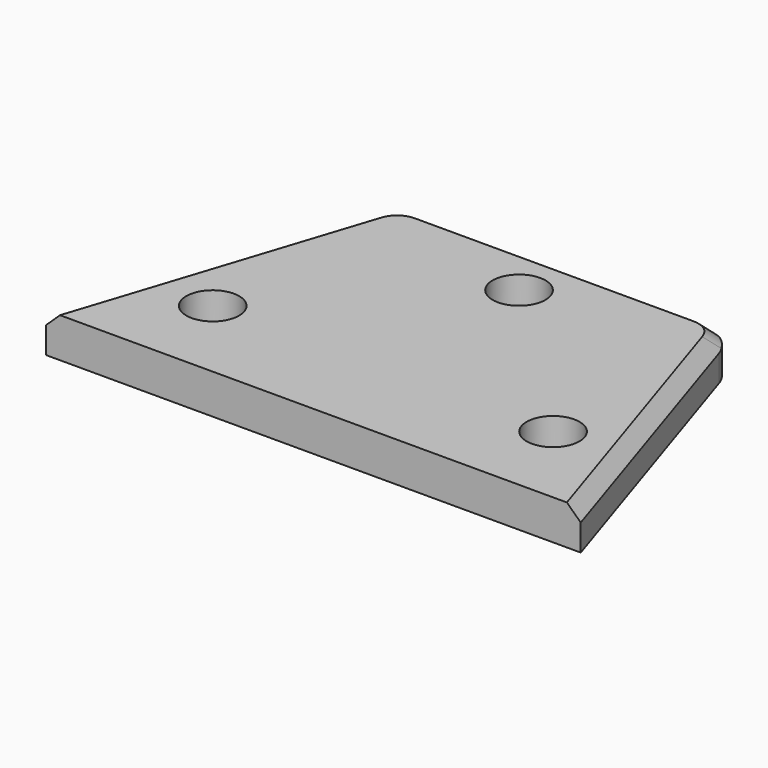
from build123d import *

# Parameters (mm, degrees)
F0_R     = 4
F1_DEPTH = 6
F2_SIZE  = 2
F3_F1_R  = 5
F3_F2_R  = 5
F3_F3_R  = 5
F3_F4_R  = 5


with BuildPart() as f1:
    # F0 (on Top) → F1 (new body)
    with BuildSketch(Plane.XY):
        Polygon((40.4508497187, -13.143277803), (25, 34.4095480118), (-25, 34.4095480118), (-40.4508497187, -13.143277803), align=None)
        with Locations((-25.7480759174, 0)):
            Circle(F0_R, mode=Mode.SUBTRACT)
        with Locations((25.7480759174, 0)):
            Circle(F0_R, mode=Mode.SUBTRACT)
        with Locations((0, 25.7480759174)):
            Circle(F0_R, mode=Mode.SUBTRACT)
    extrude(amount=F1_DEPTH)

    # F2
    f2_edges = [f1.edges().sort_by_distance(p)[0] for p in [
        (0, 34.409548, 6),
        (32.725425, 10.633135, 6),
        (-32.725425, 10.633135, 6),
    ]]
    chamfer(f2_edges, length=F2_SIZE)

    # F3: fillet of radius 5 on 4 edges, made by hand

    # F3_f1
    f3_f1_edges = [f1.edges().sort_by_distance(p)[0] for p in [
        (25, 34.4095480118, 2),
    ]]
    fillet(f3_f1_edges, radius=F3_F1_R)

    # F3_f2
    f3_f2_edges = [f1.edges().sort_by_distance(p)[0] for p in [
        (23.9265642827, 32.9320904977, 5.4774575141),
    ]]
    fillet(f3_f2_edges, radius=F3_F2_R)

    # F3_f3
    f3_f3_edges = [f1.edges().sort_by_distance(p)[0] for p in [
        (-25, 34.4095480118, 2),
    ]]
    fillet(f3_f3_edges, radius=F3_F3_R)

    # F3_f4
    f3_f4_edges = [f1.edges().sort_by_distance(p)[0] for p in [
        (-23.9265642827, 32.9320904977, 5.4774575141),
    ]]
    fillet(f3_f4_edges, radius=F3_F4_R)


solid = f1.part
